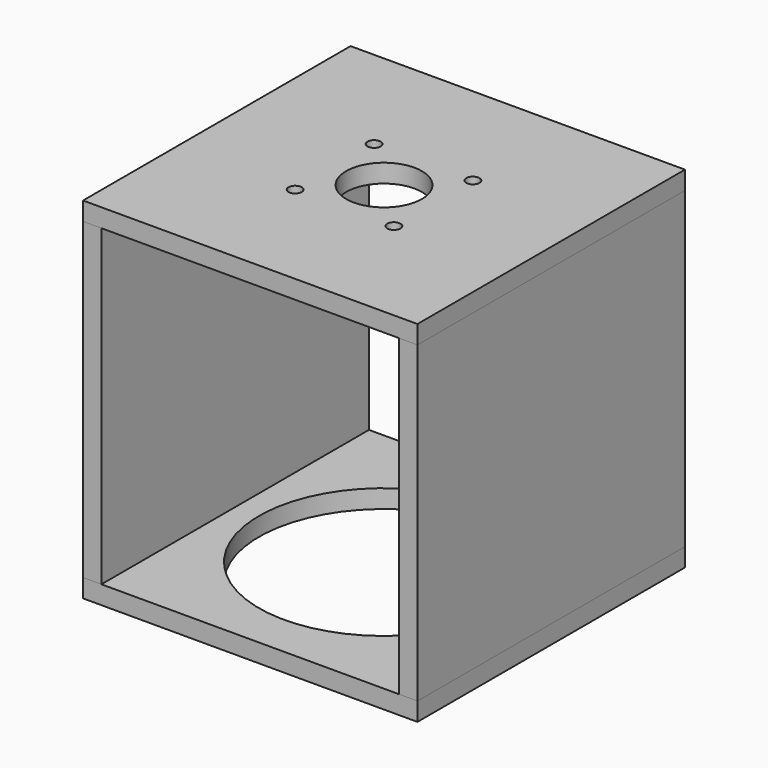
from build123d import *

# Parameters (mm, degrees)
F0_W     = 101.6
F0_H     = 101.6
F0_R     = 2
F0_R_2   = 11.5
F1_DEPTH = 5.588
F2_W     = 101.6
F2_H     = 95.25
F3_DEPTH = 5.588
F5_W     = 101.6
F5_H     = 101.6
F5_R     = 37.973
F6_DEPTH = 5.588


with BuildPart() as f1:
    # F0 (on Top) → F1 (new body)
    with BuildSketch(Plane.XY):
        Rectangle(F0_W, F0_H)
        with Locations((-15, -15)):
            Circle(F0_R, mode=Mode.SUBTRACT)
        Circle(F0_R_2, mode=Mode.SUBTRACT)
        with Locations((15, -15)):
            Circle(F0_R, mode=Mode.SUBTRACT)
        with Locations((-15, 15)):
            Circle(F0_R, mode=Mode.SUBTRACT)
        with Locations((15, 15)):
            Circle(F0_R, mode=Mode.SUBTRACT)
    extrude(amount=F1_DEPTH)


with BuildPart() as f3:
    # F2 (on face) → F3 (new body)
    with BuildSketch(Plane.YZ.offset(50.8)):
        with Locations((0, -47.625)):
            Rectangle(F2_W, F2_H)
    extrude(amount=-F3_DEPTH)


with BuildPart() as f4_1:
    # F4: instance of F3
    add(f3.part.mirror(Plane.YZ))


with BuildPart() as f6:
    # F5 (on face) → F6 (new body)
    with BuildSketch(Plane(origin=(0, 0, -95.25), x_dir=(1, 0, 0), z_dir=(0, 0, -1))):
        Rectangle(F5_W, F5_H)
        Circle(F5_R, mode=Mode.SUBTRACT)
    extrude(amount=F6_DEPTH)


solid = Compound([f1.part, f3.part, f4_1.part, f6.part])
